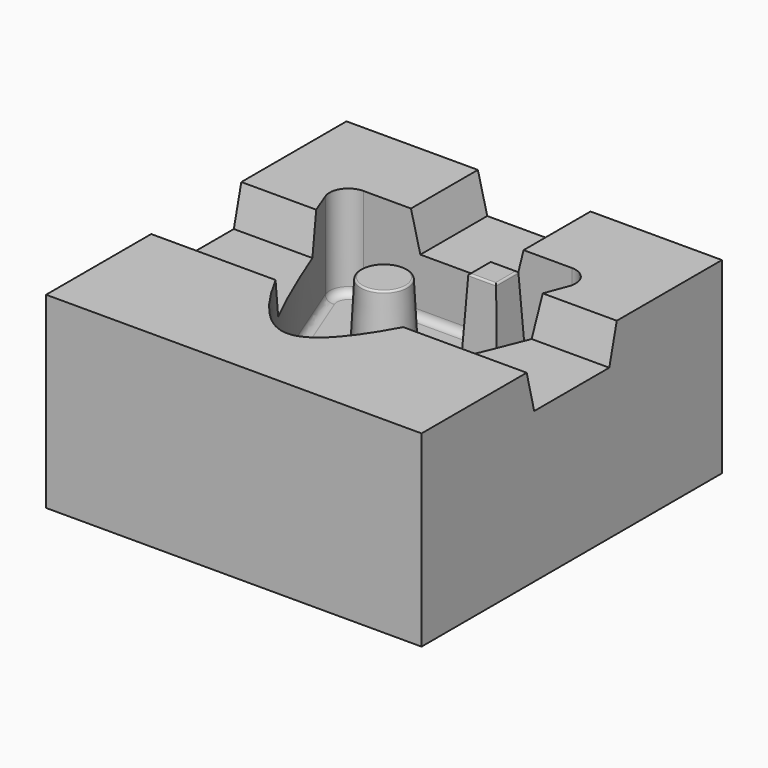
from build123d import *

# Parameters (mm, degrees)
F0_W     = 100
F0_H     = 100
F1_DEPTH = 50
F3_DEPTH = 25
F5_DEPTH = 22.275646797
F7_DEPTH = 100
F8_R     = 7.5
F8_W     = 10
F8_H     = 10
F9_DEPTH = 25
F9_TAPER = 3
F10_R    = 2
F11_R    = 0.5
F12_R    = 0.5


with BuildPart() as f1:
    # F0 (on Top) → F1 (new body)
    with BuildSketch(Plane.XY):
        Rectangle(F0_W, F0_H)
    extrude(amount=F1_DEPTH)

    # F2 (on face) → F3 (cut)
    with BuildSketch(Plane.XY.offset(50)):
        with BuildLine():
            ThreePointArc((-27.6920917798, 27.7259293121), (-31.8171440994, 25.5516150722), (-32.3544992545, 20.9196664012))
            add(Edge.make_bspline(
                [(-32.3544992545, 20.9196664012), (-23.103090057, -2.9601436233), (-0.2425590805, -61.5865364676), (23.6450097648, -2.9646096828), (32.5238265853, 20.9872745586)],
                knots=[0.0444691943, 0.0444691943, 0.0444691943, 0.0444691943, 0.5000014683, 0.9560875796, 0.9560875796, 0.9560875796, 0.9560875796], degree=3))
            ThreePointArc((32.5238265853, 20.9872745586), (31.9398334839, 25.5808897558), (27.8356444162, 27.7251799922))
            Line((27.8356444162, 27.7251799922), (-27.6920917798, 27.7259293121))
        make_face()
    extrude(amount=-F3_DEPTH, mode=Mode.SUBTRACT)

    # F4 (on face) → F5 (cut, through all)
    with BuildSketch(Plane(origin=(0, 50, 0), x_dir=(-1, 0, 0), z_dir=(0, 1, 0))):
        Polygon((15, 50), (-15, 50), (-12.5, 40), (12.5, 40), align=None)
    extrude(amount=-F5_DEPTH, mode=Mode.SUBTRACT)

    # F6 (on face) → F7 (cut)
    with BuildSketch(Plane(origin=(-50, 0, 0), x_dir=(0, -1, 0), z_dir=(-1, 0, 0))):
        Polygon((15, 50), (-15, 50), (-12.5, 40), (12.5, 40), align=None)
    extrude(amount=-F7_DEPTH, mode=Mode.SUBTRACT)

    # F8 (on face) → F9 (join)
    with BuildSketch(Plane.XY.offset(25)):
        Circle(F8_R)
        with Locations((16.3814044744, 15.9227793291)):
            Rectangle(F8_W, F8_H)
    extrude(amount=F9_DEPTH, taper=F9_TAPER)

    # F10
    f10_edges = [f1.edges().sort_by_distance(p)[0] for p in [
        (0.071776, 27.725555, 25),
        (31.939833, 25.58089, 25),
        (-31.817144, 25.551615, 25),
        (0.102186, -32.273864, 25),
        (-7.5, 0, 25),
        (11.381404, 15.922779, 25),
        (16.381404, 10.922779, 25),
        (21.381404, 15.922779, 25),
        (16.381404, 20.922779, 25),
    ]]
    fillet(f10_edges, radius=F10_R)

    # F11
    f11_edges = [f1.edges().sort_by_distance(p)[0] for p in [
        (-6.189806, 0, 50),
    ]]
    fillet(f11_edges, radius=F11_R)

    # F12
    f12_edges = [f1.edges().sort_by_distance(p)[0] for p in [
        (16.381404, 12.232974, 50),
        (12.691599, 15.922779, 50),
        (16.381404, 19.612585, 50),
        (20.07121, 15.922779, 50),
    ]]
    fillet(f12_edges, radius=F12_R)


solid = f1.part
